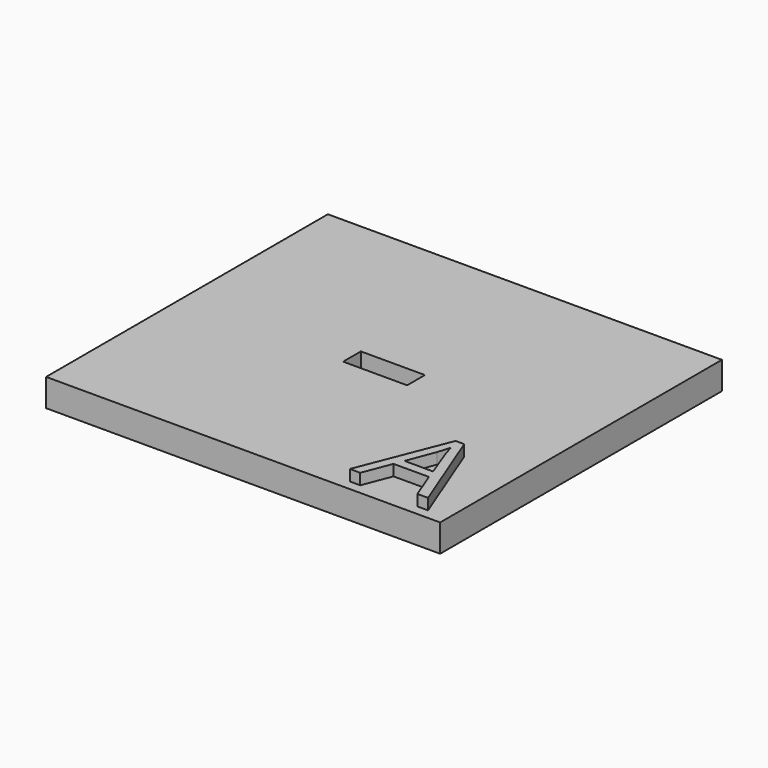
from build123d import *

# Parameters (mm, degrees)
F0_W         = 71.4546218514
F0_H         = 63.8686865568
F0_W_2       = 11.6135082208
F0_H_2       = 4.0275729261
F1_DEPTH     = 5
F2_TEXT_SIZE = 22.4127744635
F3_DEPTH     = 2


# Not quite as in the source:
# - Text() gives the source's letters only with a copy of the font that has no kerning and outlines rounded to 1/6400 em; it was checked with that copy


with BuildPart() as f1:
    # F0 (on Top) → F1 (new body)
    with BuildSketch(Plane.XY):
        Rectangle(F0_W, F0_H)
        Rectangle(F0_W_2, F0_H_2, mode=Mode.SUBTRACT)
    extrude(amount=F1_DEPTH)

    # F2 (on face) → F3 (join)
    with BuildSketch(Plane.XY.offset(5)):
        with Locations((17.8948817775, -30.114739202)):
            Text('A', F2_TEXT_SIZE, font='Open Sans', text_align=(TextAlign.LEFT, TextAlign.BOTTOM))
    extrude(amount=F3_DEPTH)


solid = f1.part
